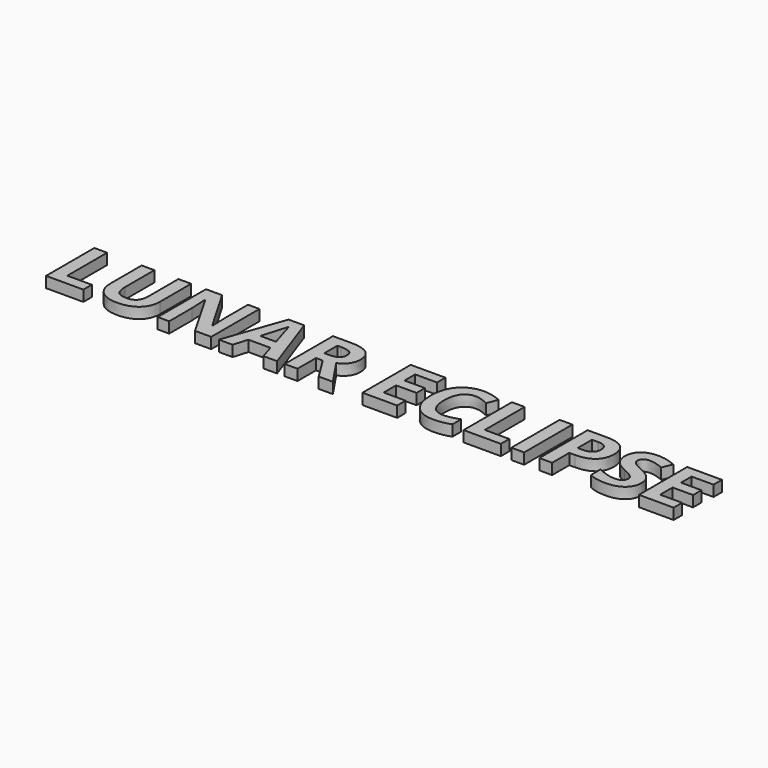
from build123d import *

# Parameters (mm, degrees)
F0_TEXT_SIZE = 38.7892062362
F1_DEPTH     = 5


# Not quite as in the source:
# - Text() gives the source's letters only with a copy of the font that has no kerning and outlines rounded to 1/6400 em; it was checked with that copy


with BuildPart() as f1:
    # F0 (on Top) → F1 (new body)
    with BuildSketch(Plane.XY):
        with Locations((-57.7563345432, 9.4044031575)):
            Text('LUNAR ECLIPSE', F0_TEXT_SIZE, font='Open Sans', font_style=FontStyle.BOLD, text_align=(TextAlign.LEFT, TextAlign.BOTTOM))
    extrude(amount=F1_DEPTH)


solid = f1.part
